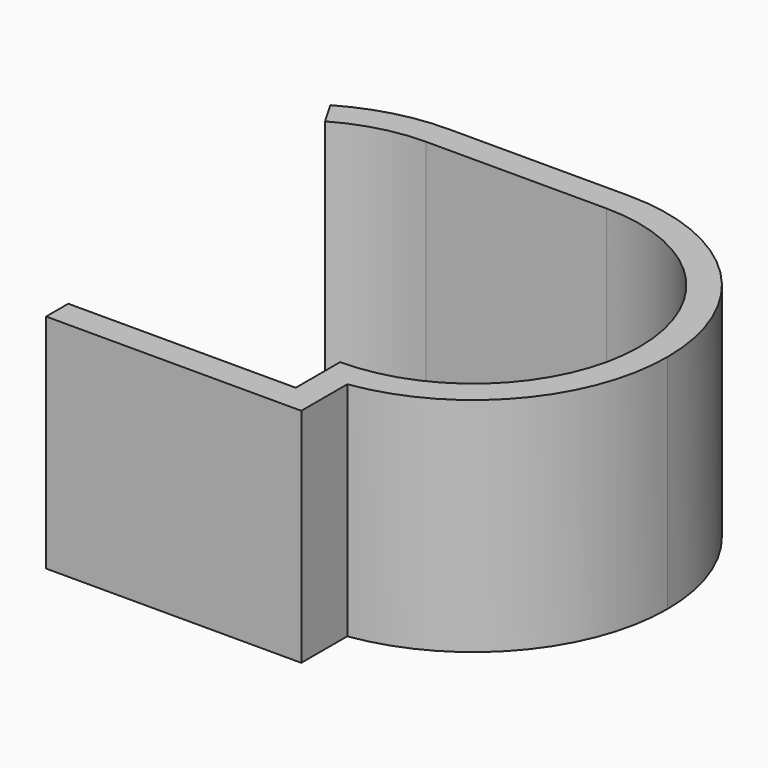
from build123d import *

# Parameters (mm, degrees)
F0_W     = 8.2
F0_H     = 1
F1_DEPTH = 8


with BuildPart() as f1:
    # F0 (on Top) → F1 (new body)
    with BuildSketch(Plane.XY):
        with Locations((-2.6644755177, -7.6461574882)):
            Rectangle(F0_W, F0_H)
        with BuildLine():
            Line((1.4355244823, -6.1461574882), (1.4355244823, -7.1461574882))
            Line((1.4355244823, -7.1461574882), (1.4355244823, -8.1461574882))
            Line((1.4355244823, -8.1461574882), (2.4355244823, -8.1461574882))
            Line((2.4355244823, -8.1461574882), (2.4355244823, -6.0743607185))
            ThreePointArc((2.4355244823, -6.0743607185), (1.9368115199, -6.1281852242), (1.4355244823, -6.1461574882))
        make_face()
        with BuildLine():
            Line((1.4355244823, -5.1461574882), (1.4355244823, -6.1461574882))
            ThreePointArc((1.4355244823, -6.1461574882), (1.9368115199, -6.1281852242), (2.4355244823, -6.0743607185))
            Line((2.4355244823, -6.0743607185), (2.4355244823, -5.1461574882))
            Line((2.4355244823, -5.1461574882), (1.4355244823, -5.1461574882))
        make_face()
        with BuildLine():
            ThreePointArc((7.4355244823, 0.8538425118), (5.6781651694, -3.3887981753), (1.4355244823, -5.1461574882))
            Line((1.4355244823, -5.1461574882), (2.4355244823, -5.1461574882))
            Line((2.4355244823, -5.1461574882), (2.4355244823, -6.0743607185))
            ThreePointArc((2.4355244823, -6.0743607185), (6.7270271044, -3.7287331832), (8.4355244823, 0.8538425118))
            ThreePointArc((8.4355244823, 0.8538425118), (6.3852719506, 5.8035899801), (1.4355244823, 7.8538425118))
            Line((1.4355244823, 7.8538425118), (1.4355244823, 6.8538425118))
            ThreePointArc((1.4355244823, 6.8538425118), (5.6781651694, 5.0964831989), (7.4355244823, 0.8538425118))
        make_face()
        with BuildLine():
            ThreePointArc((-5.0644755177, 7.8538425118), (-6.8762088334, 7.6153232958), (-8.5644755177, 6.9160203383))
            Line((-8.5644755177, 6.9160203383), (-8.0644755177, 6.0499949345))
            ThreePointArc((-8.0644755177, 6.0499949345), (-6.6173897883, 6.6493974695), (-5.0644755177, 6.8538425118))
            Line((-5.0644755177, 6.8538425118), (-5.0644755177, 7.8538425118))
        make_face()
        with BuildLine():
            Line((-1.4589242423, 6.8538425118), (1.4355244823, 6.8538425118))
            Line((1.4355244823, 6.8538425118), (1.4355244823, 7.8538425118))
            ThreePointArc((1.4355244823, 7.8538425118), (-0.2380064128, 7.6508487898), (-1.8144755177, 7.0536408956))
            ThreePointArc((-1.8144755177, 7.0536408956), (-1.6352444565, 6.956331703), (-1.4589242423, 6.8538425118))
        make_face()
        with BuildLine():
            ThreePointArc((-1.8144755177, 7.0536408956), (-3.3909446227, 7.6508487898), (-5.0644755177, 7.8538425118))
            Line((-5.0644755177, 7.8538425118), (-5.0644755177, 6.8538425118))
            Line((-5.0644755177, 6.8538425118), (-2.1700267932, 6.8538425118))
            ThreePointArc((-2.1700267932, 6.8538425118), (-1.9937065789, 6.956331703), (-1.8144755177, 7.0536408956))
        make_face()
        with BuildLine():
            Line((1.4355244823, 7.8538425118), (-5.0644755177, 7.8538425118))
            ThreePointArc((-5.0644755177, 7.8538425118), (-3.3909446227, 7.6508487898), (-1.8144755177, 7.0536408956))
            ThreePointArc((-1.8144755177, 7.0536408956), (-0.2380064128, 7.6508487898), (1.4355244823, 7.8538425118))
        make_face()
        with BuildLine():
            Line((-2.1700267932, 6.8538425118), (-1.4589242423, 6.8538425118))
            ThreePointArc((-1.4589242423, 6.8538425118), (-1.6352444565, 6.956331703), (-1.8144755177, 7.0536408956))
            ThreePointArc((-1.8144755177, 7.0536408956), (-1.9937065789, 6.956331703), (-2.1700267932, 6.8538425118))
        make_face()
    extrude(amount=F1_DEPTH)


solid = f1.part
